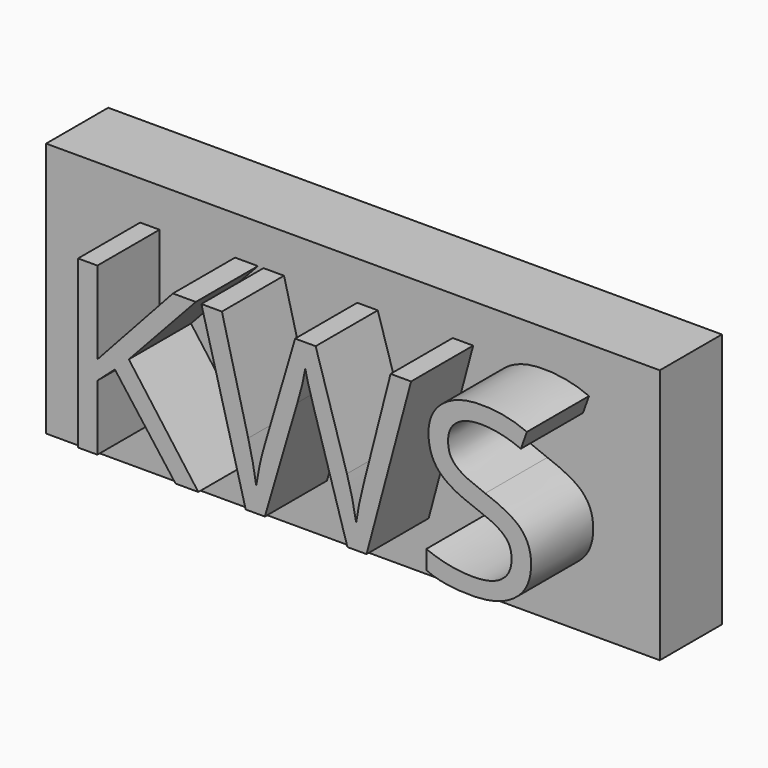
from build123d import *

# Parameters (mm, degrees)
F0_W         = 100.3812104464
F0_H         = 41.7563691735
F1_DEPTH     = 12.7
F2_TEXT_SIZE = 38.151210174
F3_DEPTH     = 12.7


# Not quite as in the source:
# - Text() gives the source's letters only with a copy of the font that has no kerning and outlines rounded to 1/6400 em; it was checked with that copy


with BuildPart() as f1:
    # F0 (on Front) → F1 (new body)
    with BuildSketch(Plane.XZ):
        with Locations((50.1906052232, 20.8781845868)):
            Rectangle(F0_W, F0_H)
    extrude(amount=F1_DEPTH)

    # F2 (on face) → F3 (join)
    with BuildSketch(Plane.XZ.offset(12.7)):
        with Locations((11.6451568902, 8.151109796)):
            Text('KWS', F2_TEXT_SIZE, font='Open Sans', text_align=(TextAlign.LEFT, TextAlign.BOTTOM))
    extrude(amount=F3_DEPTH)


solid = f1.part
